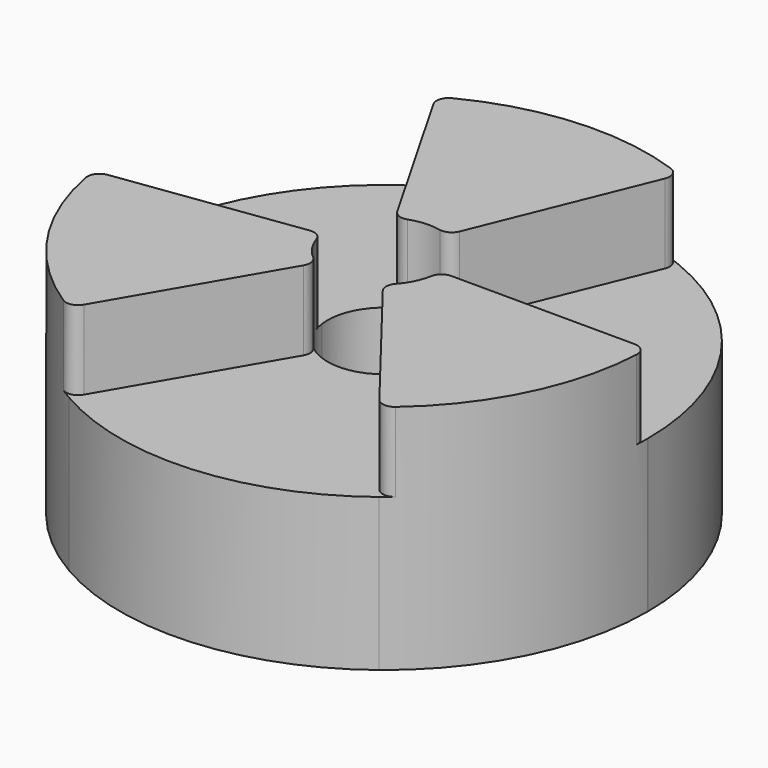
from build123d import *

# Parameters (mm, degrees)
F1_DEPTH    = 3.302
F2_DEPTH    = 6.35
F3_T1_DEPTH = 4.6338919233
F4_T1_DEPTH = 4.4582047696


# Not quite as in the source:
# - a fillet or chamfer that OpenCascade refuses, or shapes differently, is made with other operations: its cross-section is extruded or revolved along the edge and cut away or added


with BuildPart() as f1:
    # F0 (on Top) → F1 (new body)
    with BuildSketch(Plane.XY):
        with BuildLine():
            Line((0.8864303251, 2.1758656964), (4.1494522244, 10.1854037464))
            ThreePointArc((4.1494522244, 10.1854037464), (-0.7354841661, 10.9735803766), (-5.4715498037, 9.5405736717))
            Line((-5.4715498037, 9.5405736717), (-1.1688645655, 2.0381133132))
            ThreePointArc((-1.1688645655, 2.0381133132), (-0.157118442, 2.3442406116), (0.8864303251, 2.1758656964))
        make_face()
    extrude(amount=F1_DEPTH)



with BuildPart() as f1b:
    # F0 (on Top) → F1, piece 2 (new body)
    with BuildSketch(Plane.XY):
        with BuildLine():
            Line((-2.3275701308, -0.320261668), (-10.8955445044, -1.4991708351))
            ThreePointArc((-10.8955445044, -1.4991708351), (-9.1356572935, -6.1237381602), (-5.5266042645, -9.5087879639))
            Line((-5.5266042645, -9.5087879639), (-1.1806256223, -2.0313230639))
            ThreePointArc((-1.1806256223, -2.0313230639), (-1.9516127013, -1.3081888679), (-2.3275701308, -0.320261668))
        make_face()
    extrude(amount=F1_DEPTH)


with BuildPart() as f1c:
    # F0 (on Top) → F1, piece 3 (new body)
    with BuildSketch(Plane.XY):
        with BuildLine():
            ThreePointArc((6.74609228, -8.6862329113), (9.8711414597, -4.8498422164), (10.9981540682, -0.0317857078))
            Line((10.9981540682, -0.0317857078), (2.3494901878, -0.0067902494))
            ThreePointArc((2.3494901878, -0.0067902494), (2.1087311432, -1.0360517437), (1.4411398058, -1.8556040284))
            Line((1.4411398058, -1.8556040284), (6.74609228, -8.6862329113))
        make_face()
    extrude(amount=F1_DEPTH)


with BuildPart() as f1_1:
    add(f1.part)

    add(f1b.part)  # F2 merges F1b

    add(f1c.part)  # F2 merges F1c
    # F0 (on Top) → F2 (join)
    with BuildSketch(Plane.XY):
        with BuildLine():
            ThreePointArc((10.9981540682, -0.0317857078), (10.9981885171, -0.0158928705), (10.9982, 0))
            ThreePointArc((10.9982, 0), (9.1267986911, 6.136933183), (4.1494522244, 10.1854037464))
            Line((4.1494522244, 10.1854037464), (0.8864303251, 2.1758656964))
            ThreePointArc((0.8864303251, 2.1758656964), (1.9497202747, 1.3110076661), (2.3495, 0))
            ThreePointArc((2.3495, 0), (2.3494975469, -0.0033951282), (2.3494901878, -0.0067902494))
            Line((2.3494901878, -0.0067902494), (10.9981540682, -0.0317857078))
        make_face()
        with BuildLine():
            Line((0.8864303251, 2.1758656964), (4.1494522244, 10.1854037464))
            ThreePointArc((4.1494522244, 10.1854037464), (-0.7354841661, 10.9735803766), (-5.4715498037, 9.5405736717))
            Line((-5.4715498037, 9.5405736717), (-1.1688645655, 2.0381133132))
            ThreePointArc((-1.1688645655, 2.0381133132), (-0.157118442, 2.3442406116), (0.8864303251, 2.1758656964))
        make_face()
        with BuildLine():
            ThreePointArc((6.74609228, -8.6862329113), (9.8711414597, -4.8498422164), (10.9981540682, -0.0317857078))
            Line((10.9981540682, -0.0317857078), (2.3494901878, -0.0067902494))
            ThreePointArc((2.3494901878, -0.0067902494), (2.1087311432, -1.0360517437), (1.4411398058, -1.8556040284))
            Line((1.4411398058, -1.8556040284), (6.74609228, -8.6862329113))
        make_face()
        with BuildLine():
            Line((-1.1688645655, 2.0381133132), (-5.4715498037, 9.5405736717))
            ThreePointArc((-5.4715498037, 9.5405736717), (-9.8711414597, 4.8498422164), (-10.8955445044, -1.4991708351))
            Line((-10.8955445044, -1.4991708351), (-2.3275701308, -0.320261668))
            ThreePointArc((-2.3275701308, -0.320261668), (-2.1087311432, 1.0360517437), (-1.1688645655, 2.0381133132))
        make_face()
        with BuildLine():
            ThreePointArc((-5.5266042645, -9.5087879639), (0.7354841661, -10.9735803766), (6.74609228, -8.6862329113))
            Line((6.74609228, -8.6862329113), (1.4411398058, -1.8556040284))
            ThreePointArc((1.4411398058, -1.8556040284), (0.157118442, -2.3442406116), (-1.1806256223, -2.0313230639))
            Line((-1.1806256223, -2.0313230639), (-5.5266042645, -9.5087879639))
        make_face()
        with BuildLine():
            Line((-2.3275701308, -0.320261668), (-10.8955445044, -1.4991708351))
            ThreePointArc((-10.8955445044, -1.4991708351), (-9.1356572935, -6.1237381602), (-5.5266042645, -9.5087879639))
            Line((-5.5266042645, -9.5087879639), (-1.1806256223, -2.0313230639))
            ThreePointArc((-1.1806256223, -2.0313230639), (-1.9516127013, -1.3081888679), (-2.3275701308, -0.320261668))
        make_face()
    extrude(amount=-F2_DEPTH)

    # F3: fillet of radius 0.508 on 6 edges, made by hand

    # F3_s2 → F3_t1 (cut)
    with BuildSketch(Plane.XY):
        with BuildLine():
            ThreePointArc((3.9531481969, 9.7035483908), (3.9459668292, 10.1036299064), (3.6513440541, 10.3743958782))
            ThreePointArc((3.6513440541, 10.3743958782), (3.901542663, 10.2829163222), (4.1494522244, 10.1854037464))
            Line((4.1494522244, 10.1854037464), (3.9531481969, 9.7035483908))
        make_face()
        with BuildLine():
            ThreePointArc((10.9837113978, -0.5643466757), (10.8451967866, -0.1889395718), (10.4778487793, -0.0302819762))
            Line((10.4778487793, -0.0302819762), (10.9981540682, -0.0317857078))
            ThreePointArc((10.9981540682, -0.0317857078), (10.9941578867, -0.2981536556), (10.9837113978, -0.5643466757))
        make_face()
        with BuildLine():
            ThreePointArc((-5.212699429, 9.089224208), (-5.2589719244, 9.4866857122), (-5.0031171412, 9.7943464361))
            ThreePointArc((-5.0031171412, 9.7943464361), (-5.2388703034, 9.6702968509), (-5.4715498037, 9.5405736717))
            Line((-5.4715498037, 9.5405736717), (-5.212699429, 9.089224208))
        make_face()
        with BuildLine():
            ThreePointArc((7.1588183524, -8.3493546479), (6.7770167548, -8.4691224698), (6.4269453148, -8.2753009589))
            Line((6.4269453148, -8.2753009589), (6.74609228, -8.6862329113))
            ThreePointArc((6.74609228, -8.6862329113), (6.9544954285, -8.5202932212), (7.1588183524, -8.3493546479))
        make_face()
        with BuildLine():
            ThreePointArc((-5.9805942565, -9.2299997605), (-5.5862248623, -9.2977461404), (-5.2651493503, -9.0589422318))
            Line((-5.2651493503, -9.0589422318), (-5.5266042645, -9.5087879639))
            ThreePointArc((-5.5266042645, -9.5087879639), (-5.7552875833, -9.3721431953), (-5.9805942565, -9.2299997605))
        make_face()
        with BuildLine():
            ThreePointArc((-10.3800935118, -1.428247432), (-10.722983584, -1.6345074366), (-10.8101624065, -2.0250412303))
            ThreePointArc((-10.8101624065, -2.0250412303), (-10.8560380915, -1.762623101), (-10.8955445044, -1.4991708351))
            Line((-10.8955445044, -1.4991708351), (-10.3800935118, -1.428247432))
        make_face()
    extrude(amount=F3_T1_DEPTH, mode=Mode.SUBTRACT)

    # F4: fillet of radius 0.508 on 6 edges, made by hand

    # F4_s2 → F4_t1 (cut)
    with BuildSketch(Plane.XY):
        with BuildLine():
            ThreePointArc((-2.7857353042, -0.3833028373), (-2.4469491553, -0.4559663275), (-2.2335580647, -0.7289503561))
            ThreePointArc((-2.2335580647, -0.7289503561), (-2.2897006824, -0.5267077321), (-2.3275701308, -0.320261668))
            Line((-2.3275701308, -0.320261668), (-2.7857353042, -0.3833028373))
        make_face()
        with BuildLine():
            ThreePointArc((-1.5229431343, -1.7890764264), (-1.3515120564, -2.0901867434), (-1.4130231496, -2.4311741667))
            Line((-1.4130231496, -2.4311741667), (-1.1806256223, -2.0313230639))
            ThreePointArc((-1.1806256223, -2.0313230639), (-1.3572000088, -1.9178525455), (-1.5229431343, -1.7890764264))
        make_face()
        with BuildLine():
            ThreePointArc((-0.7879140674, 2.2134456561), (-1.1343987902, 2.215537146), (-1.3989470146, 2.439301027))
            Line((-1.3989470146, 2.439301027), (-1.1688645655, 2.0381133132))
            ThreePointArc((-1.1688645655, 2.0381133132), (-0.9823090207, 2.1342959584), (-0.7879140674, 2.2134456561))
        make_face()
        with BuildLine():
            ThreePointArc((0.4854895058, 2.2987932029), (0.8285961548, 2.3471032941), (1.0609176577, 2.6041689603))
            Line((1.0609176577, 2.6041689603), (0.8864303251, 2.1758656964))
            ThreePointArc((0.8864303251, 2.1758656964), (0.6887080648, 2.2462928241), (0.4854895058, 2.2987932029))
        make_face()
        with BuildLine():
            ThreePointArc((1.7248176465, -2.220866123), (1.6183530006, -1.8911369665), (1.7480685589, -1.5698428468))
            ThreePointArc((1.7480685589, -1.5698428468), (1.6009926176, -1.719585092), (1.4411398058, -1.8556040284))
            Line((1.4411398058, -1.8556040284), (1.7248176465, -2.220866123))
        make_face()
        with BuildLine():
            ThreePointArc((2.8119701642, -0.0081268603), (2.4859108466, -0.1253504027), (2.3108572018, -0.4243692296))
            ThreePointArc((2.3108572018, -0.4243692296), (2.3395090295, -0.2164434129), (2.3494901878, -0.0067902494))
            Line((2.3494901878, -0.0067902494), (2.8119701642, -0.0081268603))
        make_face()
    extrude(amount=F4_T1_DEPTH, mode=Mode.SUBTRACT)


solid = f1_1.part
